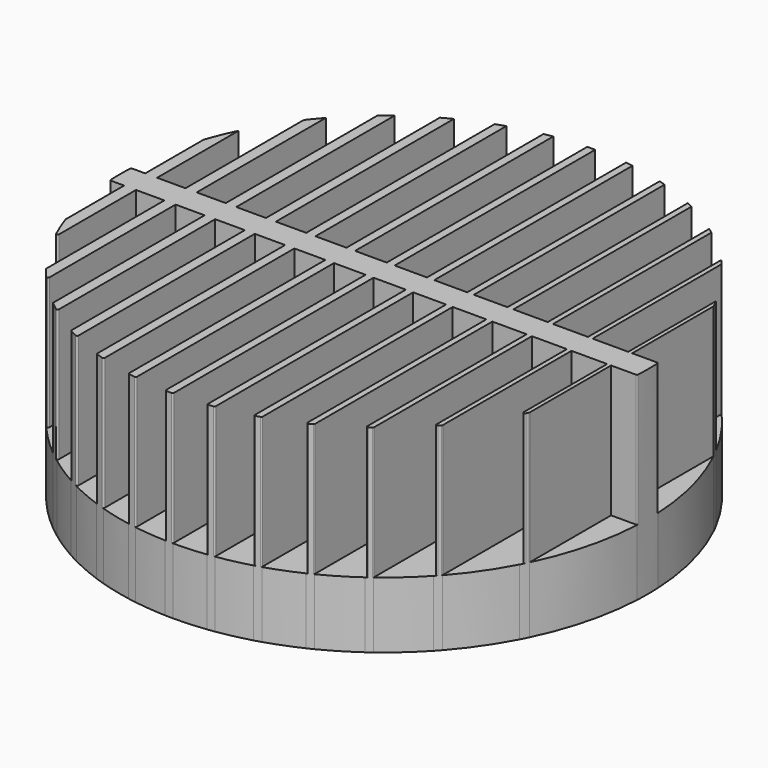
from build123d import *

# Parameters (mm, degrees)
F0_W         = 11
F0_H         = 5
F0_W_2       = 4.25
F0_W_3       = 3.25
F0_W_4       = 2.25
F0_W_5       = 3.5
F0_W_6       = 11.25
F0_W_7       = 11.5
F0_W_8       = 10.75
F0_W_9       = 4.5
F0_W_10      = 4
F0_W_11      = 3.75
F0_W_12      = 2
F0_W_13      = 13.5
F0_W_14      = 12.25
F0_W_15      = 1.75
F0_W_16      = 11.75
F0_W_17      = 13
F0_W_18      = 1.5
F0_W_19      = 2.5
F0_W_20      = 13.25
F0_W_21      = 12.75
F0_W_22      = 2.75
F0_W_23      = 12
F0_W_24      = 12.5
F0_W_25      = 3
F1_DEPTH     = 25
F2_DEPTH     = 75
F3_T1_DEPTH  = 50.2109984733
F3_T3_DEPTH  = 50.4269577712
F3_T5_DEPTH  = 53.3493232824
F3_T7_DEPTH  = 50.5880189906
F3_T9_DEPTH  = 52.5221366618
F3_T11_DEPTH = 50.7367983998
F3_T13_DEPTH = 52.0440371839
F3_T15_DEPTH = 50.8861030717
F3_T17_DEPTH = 51.7138805739
F3_T19_DEPTH = 51.0441499554
F3_T21_DEPTH = 51.4619110174
F3_T23_DEPTH = 51.2190561193
F3_T25_DEPTH = 51.2562853725
F3_T27_DEPTH = 51.4213816764
F3_T29_DEPTH = 51.0797077715
F3_T31_DEPTH = 51.6675925063
F3_T33_DEPTH = 50.921326192
F3_T35_DEPTH = 51.9875030892
F3_T37_DEPTH = 50.7731193512
F3_T39_DEPTH = 52.4451800761
F3_T41_DEPTH = 50.6275504684
F3_T43_DEPTH = 50.4743197485
F3_T45_DEPTH = 50.2878685654
F3_T47_DEPTH = 53.2195126732
F3_T49_DEPTH = 55.6061408631
F3_T51_DEPTH = 55.1888373464
F3_T53_DEPTH = 51.1948224465


# Not quite as in the source:
# - a fillet or chamfer that OpenCascade refuses, or shapes differently, is made with other operations: its cross-section is extruded or revolved along the edge and cut away or added


with BuildPart() as f1:
    # F0 (on Top) → F1 (new body)
    with BuildSketch(Plane.XY):
        with BuildLine():
            ThreePointArc((-99.8749217772, -5), (-98.1698653955, -19.0440943139), (-94.5, -32.7070328829))
            Line((-94.5, -32.7070328829), (-94.5, -5))
            Line((-94.5, -5), (-99.8749217772, -5))
        make_face()
        with BuildLine():
            Line((-94.5, -5), (-94.5, 0))
            Line((-94.5, 0), (-100, 0))
            ThreePointArc((-100, 0), (-99.9687255538, -2.5007821058), (-99.8749217772, -5))
            Line((-99.8749217772, -5), (-94.5, -5))
        make_face()
        with BuildLine():
            Line((-100, 0), (-94.5, 0))
            Line((-94.5, 0), (-94.5, 5))
            Line((-94.5, 5), (-99.8749217772, 5))
            ThreePointArc((-99.8749217772, 5), (-99.9687255538, 2.5007821058), (-100, 0))
        make_face()
        with BuildLine():
            Line((-94.5, 5), (-94.5, 32.7070328829))
            ThreePointArc((-94.5, 32.7070328829), (-98.1698653955, 19.0440943139), (-99.8749217772, 5))
            Line((-99.8749217772, 5), (-94.5, 5))
        make_face()
        with BuildLine():
            ThreePointArc((-15, -98.8685996664), (-9.0163773723, -99.5926952094), (-3, -99.9549898704))
            Line((-3, -99.9549898704), (-3, -5))
            Line((-3, -5), (-15, -5))
            Line((-15, -5), (-15, -98.8685996664))
        make_face()
        with BuildLine():
            Line((-30, 5), (-30, 95.3939201417))
            ThreePointArc((-30, 95.3939201417), (-31.7554083414, 94.8240161619), (-33.5, 94.2218127612))
            Line((-33.5, 94.2218127612), (-33.5, 5))
            Line((-33.5, 5), (-30, 5))
        make_face()
        with BuildLine():
            Line((-3, 5), (-3, 99.9549898704))
            ThreePointArc((-3, 99.9549898704), (-9.0163773723, 99.5926952094), (-15, 98.8685996664))
            Line((-15, 98.8685996664), (-15, 5))
            Line((-15, 5), (-3, 5))
        make_face()
        with BuildLine():
            ThreePointArc((12.25, -99.2468513354), (13.6263125453, -99.067268088), (15, -98.8685996664))
            Line((15, -98.8685996664), (15, -5))
            Line((15, -5), (12.25, -5))
            Line((12.25, -5), (12.25, -99.2468513354))
        make_face()
        with Locations((-69.5, -2.5)):
            Rectangle(F0_W, F0_H)
        with BuildLine():
            Line((-18.25, 5), (-18.25, 98.3205853319))
            ThreePointArc((-18.25, 98.3205853319), (-24.1693394052, 97.0352669534), (-30, 95.3939201417))
            Line((-30, 95.3939201417), (-30, 5))
            Line((-30, 5), (-18.25, 5))
        make_face()
        with Locations((-77.125, -2.5)):
            Rectangle(F0_W_2, F0_H)
        with BuildLine():
            Line((45, 5), (45, 89.3028554975))
            ThreePointArc((45, 89.3028554975), (43.878438886, 89.859237705), (42.75, 90.4015348321))
            Line((42.75, 90.4015348321), (42.75, 5))
            Line((42.75, 5), (45, 5))
        make_face()
        with Locations((-16.625, 2.5)):
            Rectangle(F0_W_3, F0_H)
        with BuildLine():
            Line((42.75, 5), (42.75, 90.4015348321))
            ThreePointArc((42.75, 90.4015348321), (36.4605485802, 93.1162091004), (30, 95.3939201417))
            Line((30, 95.3939201417), (30, 5))
            Line((30, 5), (42.75, 5))
        make_face()
        with Locations((43.875, -2.5)):
            Rectangle(F0_W_4, F0_H)
        with Locations((-31.75, -2.5)):
            Rectangle(F0_W_5, F0_H)
        with Locations((-54.375, -2.5)):
            Rectangle(F0_W_6, F0_H)
        with BuildLine():
            Line((30, 5), (30, 95.3939201417))
            ThreePointArc((30, 95.3939201417), (28.752448826, 95.7773286666), (27.5, 96.1444226151))
            Line((27.5, 96.1444226151), (27.5, 5))
            Line((27.5, 5), (30, 5))
        make_face()
        with BuildLine():
            Line((15, 5), (15, 98.8685996664))
            ThreePointArc((15, 98.8685996664), (13.6263125453, 99.067268088), (12.25, 99.2468513354))
            Line((12.25, 99.2468513354), (12.25, 5))
            Line((12.25, 5), (15, 5))
        make_face()
        with Locations((-39.25, 2.5)):
            Rectangle(F0_W_7, F0_H)
        with Locations((-84.625, 2.5)):
            Rectangle(F0_W_8, F0_H)
        with BuildLine():
            ThreePointArc((-75, -66.1437827766), (-69.7053717305, -71.7018908531), (-64, -76.8374908492))
            Line((-64, -76.8374908492), (-64, -5))
            Line((-64, -5), (-75, -5))
            Line((-75, -5), (-75, -66.1437827766))
        make_face()
        with Locations((-92.25, -2.5)):
            Rectangle(F0_W_9, F0_H)
        with BuildLine():
            ThreePointArc((45, -89.3028554975), (51.6490187326, -85.6293107759), (58, -81.4616474177))
            Line((58, -81.4616474177), (58, -5))
            Line((58, -5), (45, -5))
            Line((45, -5), (45, -89.3028554975))
        make_face()
        with Locations((-62, -2.5)):
            Rectangle(F0_W_10, F0_H)
        with BuildLine():
            ThreePointArc((15, -98.8685996664), (21.2936090213, -97.7066129535), (27.5, -96.1444226151))
            Line((27.5, -96.1444226151), (27.5, -5))
            Line((27.5, -5), (15, -5))
            Line((15, -5), (15, -98.8685996664))
        make_face()
        with Locations((-46.875, -2.5)):
            Rectangle(F0_W_11, F0_H)
        with BuildLine():
            Line((73.25, 5), (73.25, 68.0767030635))
            ThreePointArc((73.25, 68.0767030635), (66.8911943193, 74.3341652441), (60, 80))
            Line((60, 80), (60, 5))
            Line((60, 5), (73.25, 5))
        make_face()
        with BuildLine():
            ThreePointArc((-18.25, -98.3205853319), (-16.6272578896, -98.6079829176), (-15, -98.8685996664))
            Line((-15, -98.8685996664), (-15, -5))
            Line((-15, -5), (-18.25, -5))
            Line((-18.25, -5), (-18.25, -98.3205853319))
        make_face()
        with Locations((59, 2.5)):
            Rectangle(F0_W_12, F0_H)
        with Locations((81.75, 2.5)):
            Rectangle(F0_W_13, F0_H)
        with BuildLine():
            ThreePointArc((88.5, -46.559102225), (89.262354285, -45.0802851311), (90, -43.5889894354))
            Line((90, -43.5889894354), (90, -5))
            Line((90, -5), (88.5, -5))
            Line((88.5, -5), (88.5, -46.559102225))
        make_face()
        with Locations((6.125, -2.5)):
            Rectangle(F0_W_14, F0_H)
        with BuildLine():
            ThreePointArc((0, -100), (6.1365652631, -99.811535239), (12.25, -99.2468513354))
            Line((12.25, -99.2468513354), (12.25, -5))
            Line((12.25, -5), (0, -5))
            Line((0, -5), (0, -100))
        make_face()
        with BuildLine():
            Line((0, 5), (0, 100))
            ThreePointArc((0, 100), (-1.5001688165, 99.9887468344), (-3, 99.9549898704))
            Line((-3, 99.9549898704), (-3, 5))
            Line((-3, 5), (0, 5))
        make_face()
        with BuildLine():
            ThreePointArc((90, -43.5889894354), (96.8782690101, -24.7911474848), (99.8749217772, -5))
            Line((99.8749217772, -5), (90, -5))
            Line((90, -5), (90, -43.5889894354))
        make_face()
        with Locations((74.125, 2.5)):
            Rectangle(F0_W_15, F0_H)
        with BuildLine():
            Line((-79.25, 5), (-79.25, 60.9871912782))
            ThreePointArc((-79.25, 60.9871912782), (-85.0709408778, 52.5636282819), (-90, 43.5889894354))
            Line((-90, 43.5889894354), (-90, 5))
            Line((-90, 5), (-79.25, 5))
        make_face()
        with BuildLine():
            ThreePointArc((-64, -76.8374908492), (-62.0201609643, -78.4442453847), (-60, -80))
            Line((-60, -80), (-60, -5))
            Line((-60, -5), (-64, -5))
            Line((-64, -5), (-64, -76.8374908492))
        make_face()
        with BuildLine():
            Line((-48.75, 5), (-48.75, 87.3122986755))
            ThreePointArc((-48.75, 87.3122986755), (-54.4977802574, 83.845047242), (-60, 80))
            Line((-60, 80), (-60, 5))
            Line((-60, 5), (-48.75, 5))
        make_face()
        with BuildLine():
            ThreePointArc((42.75, -90.4015348321), (43.878438886, -89.859237705), (45, -89.3028554975))
            Line((45, -89.3028554975), (45, -5))
            Line((45, -5), (42.75, -5))
            Line((42.75, -5), (42.75, -90.4015348321))
        make_face()
        with BuildLine():
            ThreePointArc((60, -80), (66.8911943193, -74.3341652441), (73.25, -68.0767030635))
            Line((73.25, -68.0767030635), (73.25, -5))
            Line((73.25, -5), (60, -5))
            Line((60, -5), (60, -80))
        make_face()
        with Locations((-62, 2.5)):
            Rectangle(F0_W_10, F0_H)
        with Locations((-24.125, -2.5)):
            Rectangle(F0_W_16, F0_H)
        with BuildLine():
            ThreePointArc((58, -81.4616474177), (59.0045261255, -80.7370168925), (60, -80))
            Line((60, -80), (60, -5))
            Line((60, -5), (58, -5))
            Line((58, -5), (58, -81.4616474177))
        make_face()
        with BuildLine():
            ThreePointArc((-60, -80), (-54.4977802574, -83.845047242), (-48.75, -87.3122986755))
            Line((-48.75, -87.3122986755), (-48.75, -5))
            Line((-48.75, -5), (-60, -5))
            Line((-60, -5), (-60, -80))
        make_face()
        with Locations((51.5, -2.5)):
            Rectangle(F0_W_17, F0_H)
        with BuildLine():
            Line((27.5, 5), (27.5, 96.1444226151))
            ThreePointArc((27.5, 96.1444226151), (21.2936090213, 97.7066129535), (15, 98.8685996664))
            Line((15, 98.8685996664), (15, 5))
            Line((15, 5), (27.5, 5))
        make_face()
        with Locations((89.25, -2.5)):
            Rectangle(F0_W_18, F0_H)
        with BuildLine():
            Line((-75, 5), (-75, 66.1437827766))
            ThreePointArc((-75, 66.1437827766), (-77.1680842964, 63.6009965805), (-79.25, 60.9871912782))
            Line((-79.25, 60.9871912782), (-79.25, 5))
            Line((-79.25, 5), (-75, 5))
        make_face()
        with Locations((-39.25, -2.5)):
            Rectangle(F0_W_7, F0_H)
        with BuildLine():
            ThreePointArc((-94.5, -32.7070328829), (-92.410317306, -38.2143069464), (-90, -43.5889894354))
            Line((-90, -43.5889894354), (-90, -5))
            Line((-90, -5), (-94.5, -5))
            Line((-94.5, -5), (-94.5, -32.7070328829))
        make_face()
        with Locations((74.125, -2.5)):
            Rectangle(F0_W_15, F0_H)
        with Locations((28.75, -2.5)):
            Rectangle(F0_W_19, F0_H)
        with Locations((66.625, 2.5)):
            Rectangle(F0_W_20, F0_H)
        with Locations((-54.375, 2.5)):
            Rectangle(F0_W_6, F0_H)
        with BuildLine():
            ThreePointArc((-33.5, -94.2218127612), (-31.7554083414, -94.8240161619), (-30, -95.3939201417))
            Line((-30, -95.3939201417), (-30, -5))
            Line((-30, -5), (-33.5, -5))
            Line((-33.5, -5), (-33.5, -94.2218127612))
        make_face()
        with Locations((36.375, -2.5)):
            Rectangle(F0_W_21, F0_H)
        with Locations((66.625, -2.5)):
            Rectangle(F0_W_20, F0_H)
        with Locations((59, -2.5)):
            Rectangle(F0_W_12, F0_H)
        with BuildLine():
            Line((60, 5), (60, 80))
            ThreePointArc((60, 80), (59.0045261255, 80.7370168925), (58, 81.4616474177))
            Line((58, 81.4616474177), (58, 5))
            Line((58, 5), (60, 5))
        make_face()
        with Locations((43.875, 2.5)):
            Rectangle(F0_W_4, F0_H)
        with BuildLine():
            ThreePointArc((-45, -89.3028554975), (-39.3269822786, -91.942310526), (-33.5, -94.2218127612))
            Line((-33.5, -94.2218127612), (-33.5, -5))
            Line((-33.5, -5), (-45, -5))
            Line((-45, -5), (-45, -89.3028554975))
        make_face()
        with Locations((-46.875, 2.5)):
            Rectangle(F0_W_11, F0_H)
        with BuildLine():
            Line((-60, 5), (-60, 80))
            ThreePointArc((-60, 80), (-62.0201609643, 78.4442453847), (-64, 76.8374908492))
            Line((-64, 76.8374908492), (-64, 5))
            Line((-64, 5), (-60, 5))
        make_face()
        with BuildLine():
            ThreePointArc((-90, -43.5889894354), (-85.0709408778, -52.5636282819), (-79.25, -60.9871912782))
            Line((-79.25, -60.9871912782), (-79.25, -5))
            Line((-79.25, -5), (-90, -5))
            Line((-90, -5), (-90, -43.5889894354))
        make_face()
        with Locations((-16.625, -2.5)):
            Rectangle(F0_W_3, F0_H)
        with BuildLine():
            Line((12.25, 5), (12.25, 99.2468513354))
            ThreePointArc((12.25, 99.2468513354), (6.1365652631, 99.811535239), (0, 100))
            Line((0, 100), (0, 5))
            Line((0, 5), (12.25, 5))
        make_face()
        with BuildLine():
            Line((90, 5), (99.8749217772, 5))
            ThreePointArc((99.8749217772, 5), (96.8782690101, 24.7911474848), (90, 43.5889894354))
            Line((90, 43.5889894354), (90, 5))
        make_face()
        with Locations((-84.625, -2.5)):
            Rectangle(F0_W_8, F0_H)
        with Locations((-69.5, 2.5)):
            Rectangle(F0_W, F0_H)
        with BuildLine():
            ThreePointArc((27.5, -96.1444226151), (28.752448826, -95.7773286666), (30, -95.3939201417))
            Line((30, -95.3939201417), (30, -5))
            Line((30, -5), (27.5, -5))
            Line((27.5, -5), (27.5, -96.1444226151))
        make_face()
        with BuildLine():
            ThreePointArc((-48.75, -87.3122986755), (-46.8855649866, -88.3274804117), (-45, -89.3028554975))
            Line((-45, -89.3028554975), (-45, -5))
            Line((-45, -5), (-48.75, -5))
            Line((-48.75, -5), (-48.75, -87.3122986755))
        make_face()
        with BuildLine():
            Line((90, 5), (90, 43.5889894354))
            ThreePointArc((90, 43.5889894354), (89.262354285, 45.0802851311), (88.5, 46.559102225))
            Line((88.5, 46.559102225), (88.5, 5))
            Line((88.5, 5), (90, 5))
        make_face()
        with Locations((-77.125, 2.5)):
            Rectangle(F0_W_2, F0_H)
        with Locations((13.625, 2.5)):
            Rectangle(F0_W_22, F0_H)
        with BuildLine():
            Line((-33.5, 5), (-33.5, 94.2218127612))
            ThreePointArc((-33.5, 94.2218127612), (-39.3269822786, 91.942310526), (-45, 89.3028554975))
            Line((-45, 89.3028554975), (-45, 5))
            Line((-45, 5), (-33.5, 5))
        make_face()
        with Locations((-24.125, 2.5)):
            Rectangle(F0_W_16, F0_H)
        with Locations((-9, -2.5)):
            Rectangle(F0_W_23, F0_H)
        with Locations((21.25, -2.5)):
            Rectangle(F0_W_24, F0_H)
        with BuildLine():
            Line((-15, 5), (-15, 98.8685996664))
            ThreePointArc((-15, 98.8685996664), (-16.6272578896, 98.6079829176), (-18.25, 98.3205853319))
            Line((-18.25, 98.3205853319), (-18.25, 5))
            Line((-18.25, 5), (-15, 5))
        make_face()
        with BuildLine():
            ThreePointArc((99.8749217772, -5), (99.9687255538, -2.5007821058), (100, 0))
            Line((100, 0), (90, 0))
            Line((90, 0), (90, -5))
            Line((90, -5), (99.8749217772, -5))
        make_face()
        with Locations((36.375, 2.5)):
            Rectangle(F0_W_21, F0_H)
        with BuildLine():
            ThreePointArc((75, -66.1437827766), (82.3343939558, -56.7542736005), (88.5, -46.559102225))
            Line((88.5, -46.559102225), (88.5, -5))
            Line((88.5, -5), (75, -5))
            Line((75, -5), (75, -66.1437827766))
        make_face()
        with Locations((6.125, 2.5)):
            Rectangle(F0_W_14, F0_H)
        with Locations((81.75, -2.5)):
            Rectangle(F0_W_13, F0_H)
        with Locations((13.625, -2.5)):
            Rectangle(F0_W_22, F0_H)
        with BuildLine():
            Line((90, 0), (100, 0))
            ThreePointArc((100, 0), (99.9687255538, 2.5007821058), (99.8749217772, 5))
            Line((99.8749217772, 5), (90, 5))
            Line((90, 5), (90, 0))
        make_face()
        with Locations((28.75, 2.5)):
            Rectangle(F0_W_19, F0_H)
        with BuildLine():
            Line((-64, 5), (-64, 76.8374908492))
            ThreePointArc((-64, 76.8374908492), (-69.7053717305, 71.7018908531), (-75, 66.1437827766))
            Line((-75, 66.1437827766), (-75, 5))
            Line((-75, 5), (-64, 5))
        make_face()
        with Locations((-92.25, 2.5)):
            Rectangle(F0_W_9, F0_H)
        with BuildLine():
            Line((88.5, 5), (88.5, 46.559102225))
            ThreePointArc((88.5, 46.559102225), (82.3343939558, 56.7542736005), (75, 66.1437827766))
            Line((75, 66.1437827766), (75, 5))
            Line((75, 5), (88.5, 5))
        make_face()
        with BuildLine():
            Line((-45, 5), (-45, 89.3028554975))
            ThreePointArc((-45, 89.3028554975), (-46.8855649866, 88.3274804117), (-48.75, 87.3122986755))
            Line((-48.75, 87.3122986755), (-48.75, 5))
            Line((-48.75, 5), (-45, 5))
        make_face()
        with BuildLine():
            ThreePointArc((30, -95.3939201417), (36.4605485802, -93.1162091004), (42.75, -90.4015348321))
            Line((42.75, -90.4015348321), (42.75, -5))
            Line((42.75, -5), (30, -5))
            Line((30, -5), (30, -95.3939201417))
        make_face()
        with Locations((-31.75, 2.5)):
            Rectangle(F0_W_5, F0_H)
        with BuildLine():
            ThreePointArc((-79.25, -60.9871912782), (-77.1680842964, -63.6009965805), (-75, -66.1437827766))
            Line((-75, -66.1437827766), (-75, -5))
            Line((-75, -5), (-79.25, -5))
            Line((-79.25, -5), (-79.25, -60.9871912782))
        make_face()
        with BuildLine():
            Line((-90, 5), (-90, 43.5889894354))
            ThreePointArc((-90, 43.5889894354), (-92.410317306, 38.2143069464), (-94.5, 32.7070328829))
            Line((-94.5, 32.7070328829), (-94.5, 5))
            Line((-94.5, 5), (-90, 5))
        make_face()
        with Locations((21.25, 2.5)):
            Rectangle(F0_W_24, F0_H)
        with BuildLine():
            Line((58, 5), (58, 81.4616474177))
            ThreePointArc((58, 81.4616474177), (51.6490187326, 85.6293107759), (45, 89.3028554975))
            Line((45, 89.3028554975), (45, 5))
            Line((45, 5), (58, 5))
        make_face()
        with Locations((89.25, 2.5)):
            Rectangle(F0_W_18, F0_H)
        with BuildLine():
            Line((75, 5), (75, 66.1437827766))
            ThreePointArc((75, 66.1437827766), (74.1313002058, 67.1159469112), (73.25, 68.0767030635))
            Line((73.25, 68.0767030635), (73.25, 5))
            Line((73.25, 5), (75, 5))
        make_face()
        with Locations((-9, 2.5)):
            Rectangle(F0_W_23, F0_H)
        with BuildLine():
            ThreePointArc((-30, -95.3939201417), (-24.1693394052, -97.0352669534), (-18.25, -98.3205853319))
            Line((-18.25, -98.3205853319), (-18.25, -5))
            Line((-18.25, -5), (-30, -5))
            Line((-30, -5), (-30, -95.3939201417))
        make_face()
        with BuildLine():
            ThreePointArc((73.25, -68.0767030635), (74.1313002058, -67.1159469112), (75, -66.1437827766))
            Line((75, -66.1437827766), (75, -5))
            Line((75, -5), (73.25, -5))
            Line((73.25, -5), (73.25, -68.0767030635))
        make_face()
        with BuildLine():
            ThreePointArc((-3, -99.9549898704), (-1.5001688165, -99.9887468344), (0, -100))
            Line((0, -100), (0, -5))
            Line((0, -5), (-3, -5))
            Line((-3, -5), (-3, -99.9549898704))
        make_face()
        with Locations((51.5, 2.5)):
            Rectangle(F0_W_17, F0_H)
        with Locations((-1.5, 2.5)):
            Rectangle(F0_W_25, F0_H)
        with Locations((-1.5, -2.5)):
            Rectangle(F0_W_25, F0_H)
    extrude(amount=F1_DEPTH)

    # F0 (on Top) → F2 (join)
    with BuildSketch(Plane.XY):
        with BuildLine():
            ThreePointArc((99.8749217772, -5), (99.9687255538, -2.5007821058), (100, 0))
            Line((100, 0), (90, 0))
            Line((90, 0), (90, -5))
            Line((90, -5), (99.8749217772, -5))
        make_face()
        with BuildLine():
            Line((90, 0), (100, 0))
            ThreePointArc((100, 0), (99.9687255538, 2.5007821058), (99.8749217772, 5))
            Line((99.8749217772, 5), (90, 5))
            Line((90, 5), (90, 0))
        make_face()
        with Locations((89.25, 2.5)):
            Rectangle(F0_W_18, F0_H)
        with BuildLine():
            Line((90, 5), (90, 43.5889894354))
            ThreePointArc((90, 43.5889894354), (89.262354285, 45.0802851311), (88.5, 46.559102225))
            Line((88.5, 46.559102225), (88.5, 5))
            Line((88.5, 5), (90, 5))
        make_face()
        with Locations((81.75, 2.5)):
            Rectangle(F0_W_13, F0_H)
        with Locations((81.75, -2.5)):
            Rectangle(F0_W_13, F0_H)
        with Locations((89.25, -2.5)):
            Rectangle(F0_W_18, F0_H)
        with BuildLine():
            ThreePointArc((88.5, -46.559102225), (89.262354285, -45.0802851311), (90, -43.5889894354))
            Line((90, -43.5889894354), (90, -5))
            Line((90, -5), (88.5, -5))
            Line((88.5, -5), (88.5, -46.559102225))
        make_face()
        with Locations((74.125, -2.5)):
            Rectangle(F0_W_15, F0_H)
        with BuildLine():
            ThreePointArc((73.25, -68.0767030635), (74.1313002058, -67.1159469112), (75, -66.1437827766))
            Line((75, -66.1437827766), (75, -5))
            Line((75, -5), (73.25, -5))
            Line((73.25, -5), (73.25, -68.0767030635))
        make_face()
        with Locations((74.125, 2.5)):
            Rectangle(F0_W_15, F0_H)
        with Locations((66.625, 2.5)):
            Rectangle(F0_W_20, F0_H)
        with Locations((66.625, -2.5)):
            Rectangle(F0_W_20, F0_H)
        with BuildLine():
            Line((75, 5), (75, 66.1437827766))
            ThreePointArc((75, 66.1437827766), (74.1313002058, 67.1159469112), (73.25, 68.0767030635))
            Line((73.25, 68.0767030635), (73.25, 5))
            Line((73.25, 5), (75, 5))
        make_face()
        with Locations((59, 2.5)):
            Rectangle(F0_W_12, F0_H)
        with BuildLine():
            Line((60, 5), (60, 80))
            ThreePointArc((60, 80), (59.0045261255, 80.7370168925), (58, 81.4616474177))
            Line((58, 81.4616474177), (58, 5))
            Line((58, 5), (60, 5))
        make_face()
        with Locations((51.5, 2.5)):
            Rectangle(F0_W_17, F0_H)
        with Locations((51.5, -2.5)):
            Rectangle(F0_W_17, F0_H)
        with Locations((59, -2.5)):
            Rectangle(F0_W_12, F0_H)
        with BuildLine():
            ThreePointArc((58, -81.4616474177), (59.0045261255, -80.7370168925), (60, -80))
            Line((60, -80), (60, -5))
            Line((60, -5), (58, -5))
            Line((58, -5), (58, -81.4616474177))
        make_face()
        with Locations((43.875, -2.5)):
            Rectangle(F0_W_4, F0_H)
        with Locations((43.875, 2.5)):
            Rectangle(F0_W_4, F0_H)
        with BuildLine():
            Line((45, 5), (45, 89.3028554975))
            ThreePointArc((45, 89.3028554975), (43.878438886, 89.859237705), (42.75, 90.4015348321))
            Line((42.75, 90.4015348321), (42.75, 5))
            Line((42.75, 5), (45, 5))
        make_face()
        with Locations((36.375, 2.5)):
            Rectangle(F0_W_21, F0_H)
        with Locations((36.375, -2.5)):
            Rectangle(F0_W_21, F0_H)
        with BuildLine():
            ThreePointArc((42.75, -90.4015348321), (43.878438886, -89.859237705), (45, -89.3028554975))
            Line((45, -89.3028554975), (45, -5))
            Line((45, -5), (42.75, -5))
            Line((42.75, -5), (42.75, -90.4015348321))
        make_face()
        with Locations((28.75, -2.5)):
            Rectangle(F0_W_19, F0_H)
        with Locations((28.75, 2.5)):
            Rectangle(F0_W_19, F0_H)
        with Locations((21.25, 2.5)):
            Rectangle(F0_W_24, F0_H)
        with Locations((21.25, -2.5)):
            Rectangle(F0_W_24, F0_H)
        with BuildLine():
            Line((30, 5), (30, 95.3939201417))
            ThreePointArc((30, 95.3939201417), (28.752448826, 95.7773286666), (27.5, 96.1444226151))
            Line((27.5, 96.1444226151), (27.5, 5))
            Line((27.5, 5), (30, 5))
        make_face()
        with BuildLine():
            ThreePointArc((27.5, -96.1444226151), (28.752448826, -95.7773286666), (30, -95.3939201417))
            Line((30, -95.3939201417), (30, -5))
            Line((30, -5), (27.5, -5))
            Line((27.5, -5), (27.5, -96.1444226151))
        make_face()
        with Locations((13.625, -2.5)):
            Rectangle(F0_W_22, F0_H)
        with Locations((13.625, 2.5)):
            Rectangle(F0_W_22, F0_H)
        with Locations((6.125, 2.5)):
            Rectangle(F0_W_14, F0_H)
        with Locations((6.125, -2.5)):
            Rectangle(F0_W_14, F0_H)
        with BuildLine():
            Line((15, 5), (15, 98.8685996664))
            ThreePointArc((15, 98.8685996664), (13.6263125453, 99.067268088), (12.25, 99.2468513354))
            Line((12.25, 99.2468513354), (12.25, 5))
            Line((12.25, 5), (15, 5))
        make_face()
        with BuildLine():
            ThreePointArc((12.25, -99.2468513354), (13.6263125453, -99.067268088), (15, -98.8685996664))
            Line((15, -98.8685996664), (15, -5))
            Line((15, -5), (12.25, -5))
            Line((12.25, -5), (12.25, -99.2468513354))
        make_face()
        with Locations((-1.5, -2.5)):
            Rectangle(F0_W_25, F0_H)
        with Locations((-9, -2.5)):
            Rectangle(F0_W_23, F0_H)
        with Locations((-9, 2.5)):
            Rectangle(F0_W_23, F0_H)
        with Locations((-1.5, 2.5)):
            Rectangle(F0_W_25, F0_H)
        with BuildLine():
            Line((0, 5), (0, 100))
            ThreePointArc((0, 100), (-1.5001688165, 99.9887468344), (-3, 99.9549898704))
            Line((-3, 99.9549898704), (-3, 5))
            Line((-3, 5), (0, 5))
        make_face()
        with BuildLine():
            ThreePointArc((-3, -99.9549898704), (-1.5001688165, -99.9887468344), (0, -100))
            Line((0, -100), (0, -5))
            Line((0, -5), (-3, -5))
            Line((-3, -5), (-3, -99.9549898704))
        make_face()
        with Locations((-16.625, -2.5)):
            Rectangle(F0_W_3, F0_H)
        with BuildLine():
            ThreePointArc((-18.25, -98.3205853319), (-16.6272578896, -98.6079829176), (-15, -98.8685996664))
            Line((-15, -98.8685996664), (-15, -5))
            Line((-15, -5), (-18.25, -5))
            Line((-18.25, -5), (-18.25, -98.3205853319))
        make_face()
        with Locations((-24.125, -2.5)):
            Rectangle(F0_W_16, F0_H)
        with Locations((-24.125, 2.5)):
            Rectangle(F0_W_16, F0_H)
        with Locations((-16.625, 2.5)):
            Rectangle(F0_W_3, F0_H)
        with BuildLine():
            Line((-15, 5), (-15, 98.8685996664))
            ThreePointArc((-15, 98.8685996664), (-16.6272578896, 98.6079829176), (-18.25, 98.3205853319))
            Line((-18.25, 98.3205853319), (-18.25, 5))
            Line((-18.25, 5), (-15, 5))
        make_face()
        with BuildLine():
            Line((-30, 5), (-30, 95.3939201417))
            ThreePointArc((-30, 95.3939201417), (-31.7554083414, 94.8240161619), (-33.5, 94.2218127612))
            Line((-33.5, 94.2218127612), (-33.5, 5))
            Line((-33.5, 5), (-30, 5))
        make_face()
        with Locations((-31.75, 2.5)):
            Rectangle(F0_W_5, F0_H)
        with Locations((-39.25, 2.5)):
            Rectangle(F0_W_7, F0_H)
        with Locations((-39.25, -2.5)):
            Rectangle(F0_W_7, F0_H)
        with Locations((-31.75, -2.5)):
            Rectangle(F0_W_5, F0_H)
        with BuildLine():
            ThreePointArc((-33.5, -94.2218127612), (-31.7554083414, -94.8240161619), (-30, -95.3939201417))
            Line((-30, -95.3939201417), (-30, -5))
            Line((-30, -5), (-33.5, -5))
            Line((-33.5, -5), (-33.5, -94.2218127612))
        make_face()
        with Locations((-46.875, -2.5)):
            Rectangle(F0_W_11, F0_H)
        with BuildLine():
            ThreePointArc((-48.75, -87.3122986755), (-46.8855649866, -88.3274804117), (-45, -89.3028554975))
            Line((-45, -89.3028554975), (-45, -5))
            Line((-45, -5), (-48.75, -5))
            Line((-48.75, -5), (-48.75, -87.3122986755))
        make_face()
        with Locations((-54.375, -2.5)):
            Rectangle(F0_W_6, F0_H)
        with Locations((-46.875, 2.5)):
            Rectangle(F0_W_11, F0_H)
        with BuildLine():
            Line((-45, 5), (-45, 89.3028554975))
            ThreePointArc((-45, 89.3028554975), (-46.8855649866, 88.3274804117), (-48.75, 87.3122986755))
            Line((-48.75, 87.3122986755), (-48.75, 5))
            Line((-48.75, 5), (-45, 5))
        make_face()
        with Locations((-54.375, 2.5)):
            Rectangle(F0_W_6, F0_H)
        with Locations((-62, 2.5)):
            Rectangle(F0_W_10, F0_H)
        with Locations((-69.5, 2.5)):
            Rectangle(F0_W, F0_H)
        with Locations((-62, -2.5)):
            Rectangle(F0_W_10, F0_H)
        with BuildLine():
            ThreePointArc((-64, -76.8374908492), (-62.0201609643, -78.4442453847), (-60, -80))
            Line((-60, -80), (-60, -5))
            Line((-60, -5), (-64, -5))
            Line((-64, -5), (-64, -76.8374908492))
        make_face()
        with BuildLine():
            Line((-60, 5), (-60, 80))
            ThreePointArc((-60, 80), (-62.0201609643, 78.4442453847), (-64, 76.8374908492))
            Line((-64, 76.8374908492), (-64, 5))
            Line((-64, 5), (-60, 5))
        make_face()
        with Locations((-77.125, 2.5)):
            Rectangle(F0_W_2, F0_H)
        with Locations((-84.625, 2.5)):
            Rectangle(F0_W_8, F0_H)
        with Locations((-69.5, -2.5)):
            Rectangle(F0_W, F0_H)
        with Locations((-77.125, -2.5)):
            Rectangle(F0_W_2, F0_H)
        with BuildLine():
            ThreePointArc((-79.25, -60.9871912782), (-77.1680842964, -63.6009965805), (-75, -66.1437827766))
            Line((-75, -66.1437827766), (-75, -5))
            Line((-75, -5), (-79.25, -5))
            Line((-79.25, -5), (-79.25, -60.9871912782))
        make_face()
        with BuildLine():
            Line((-75, 5), (-75, 66.1437827766))
            ThreePointArc((-75, 66.1437827766), (-77.1680842964, 63.6009965805), (-79.25, 60.9871912782))
            Line((-79.25, 60.9871912782), (-79.25, 5))
            Line((-79.25, 5), (-75, 5))
        make_face()
        with Locations((-84.625, -2.5)):
            Rectangle(F0_W_8, F0_H)
        with Locations((-92.25, 2.5)):
            Rectangle(F0_W_9, F0_H)
        with BuildLine():
            Line((-90, 5), (-90, 43.5889894354))
            ThreePointArc((-90, 43.5889894354), (-92.410317306, 38.2143069464), (-94.5, 32.7070328829))
            Line((-94.5, 32.7070328829), (-94.5, 5))
            Line((-94.5, 5), (-90, 5))
        make_face()
        with BuildLine():
            Line((-100, 0), (-94.5, 0))
            Line((-94.5, 0), (-94.5, 5))
            Line((-94.5, 5), (-99.8749217772, 5))
            ThreePointArc((-99.8749217772, 5), (-99.9687255538, 2.5007821058), (-100, 0))
        make_face()
        with BuildLine():
            Line((-94.5, -5), (-94.5, 0))
            Line((-94.5, 0), (-100, 0))
            ThreePointArc((-100, 0), (-99.9687255538, -2.5007821058), (-99.8749217772, -5))
            Line((-99.8749217772, -5), (-94.5, -5))
        make_face()
        with Locations((-92.25, -2.5)):
            Rectangle(F0_W_9, F0_H)
        with BuildLine():
            ThreePointArc((-94.5, -32.7070328829), (-92.410317306, -38.2143069464), (-90, -43.5889894354))
            Line((-90, -43.5889894354), (-90, -5))
            Line((-90, -5), (-94.5, -5))
            Line((-94.5, -5), (-94.5, -32.7070328829))
        make_face()
    extrude(amount=F2_DEPTH)

    # F3: fillet of radius 0.5 on 30 edges, made by hand

    # F3_s2 → F3_t1 (cut)
    with BuildSketch(Plane.XY.offset(25)):
        with BuildLine():
            ThreePointArc((-94.472361809, -32.7867786496), (-94.493042039, -32.7059684458), (-94.5, -32.6228447564))
            Line((-94.5, -32.6228447564), (-94.5, -32.7070328829))
            ThreePointArc((-94.5, -32.7070328829), (-94.4861893176, -32.7469086821), (-94.472361809, -32.7867786496))
        make_face()
    extrude(amount=F3_T1_DEPTH, mode=Mode.SUBTRACT)

    # F3_s4 → F3_t3 (cut)
    with BuildSketch(Plane.XY.offset(25)):
        with BuildLine():
            ThreePointArc((-79.1457286432, -61.122447902), (-79.223214709, -60.9782910408), (-79.25, -60.8168356625))
            Line((-79.25, -60.8168356625), (-79.25, -60.9871912782))
            ThreePointArc((-79.25, -60.9871912782), (-79.197893196, -61.0548418498), (-79.1457286432, -61.122447902))
        make_face()
    extrude(amount=F3_T3_DEPTH, mode=Mode.SUBTRACT)

    # F3_s6 → F3_t5 (cut)
    with BuildSketch(Plane.XY.offset(25)):
        with BuildLine():
            ThreePointArc((-75.8793969849, -65.1330723458), (-75.3263602759, -65.2762878285), (-75, -64.8074069841))
            Line((-75, -64.8074069841), (-75, -66.1437827766))
            ThreePointArc((-75, -66.1437827766), (-75.4413911094, -65.6399002701), (-75.8793969849, -65.1330723458))
        make_face()
    extrude(amount=F3_T5_DEPTH, mode=Mode.SUBTRACT)

    # F3_s8 → F3_t7 (cut)
    with BuildSketch(Plane.XY.offset(25)):
        with BuildLine():
            ThreePointArc((-63.8190954774, -76.9878110641), (-63.9525194685, -76.8155363703), (-64, -76.6028720088))
            Line((-64, -76.6028720088), (-64, -76.8374908492))
            ThreePointArc((-64, -76.8374908492), (-63.9095919343, -76.9127041443), (-63.8190954774, -76.9878110641))
        make_face()
    extrude(amount=F3_T7_DEPTH, mode=Mode.SUBTRACT)

    # F3_s10 → F3_t9 (cut)
    with BuildSketch(Plane.XY.offset(25)):
        with BuildLine():
            ThreePointArc((-60.8040201005, -79.3906237513), (-60.2786519147, -79.4420064722), (-60, -78.9936706325))
            Line((-60, -78.9936706325), (-60, -80))
            ThreePointArc((-60, -80), (-60.4027785202, -79.6963258064), (-60.8040201005, -79.3906237513))
        make_face()
    extrude(amount=F3_T9_DEPTH, mode=Mode.SUBTRACT)

    # F3_s12 → F3_t11 (cut)
    with BuildSketch(Plane.XY.offset(25)):
        with BuildLine():
            ThreePointArc((-48.4924623116, -87.4555950123), (-48.6808312638, -87.2720578935), (-48.75, -87.0183170373))
            Line((-48.75, -87.0183170373), (-48.75, -87.3122986755))
            ThreePointArc((-48.75, -87.3122986755), (-48.6212839461, -87.3840417207), (-48.4924623116, -87.4555950123))
        make_face()
    extrude(amount=F3_T11_DEPTH, mode=Mode.SUBTRACT)

    # F3_s14 → F3_t13 (cut)
    with BuildSketch(Plane.XY.offset(25)):
        with BuildLine():
            ThreePointArc((-45.7286432161, -88.9319469573), (-45.2395404139, -88.9140902263), (-45, -88.4872872225))
            Line((-45, -88.4872872225), (-45, -89.3028554975))
            ThreePointArc((-45, -89.3028554975), (-45.364700685, -89.1181459174), (-45.7286432161, -88.9319469573))
        make_face()
    extrude(amount=F3_T13_DEPTH, mode=Mode.SUBTRACT)

    # F3_s16 → F3_t15 (cut)
    with BuildSketch(Plane.XY.offset(25)):
        with BuildLine():
            ThreePointArc((-33.1658291457, -94.3399585387), (-33.4079917725, -94.1572963103), (-33.5, -93.868258746))
            Line((-33.5, -93.868258746), (-33.5, -94.2218127612))
            ThreePointArc((-33.5, -94.2218127612), (-33.3329669176, -94.2810337049), (-33.1658291457, -94.3399585387))
        make_face()
    extrude(amount=F3_T15_DEPTH, mode=Mode.SUBTRACT)

    # F3_s18 → F3_t17 (cut)
    with BuildSketch(Plane.XY.offset(25)):
        with BuildLine():
            ThreePointArc((-30.6532663317, -95.1860140105), (-30.2055795233, -95.114208405), (-30, -94.7100839404))
            Line((-30, -94.7100839404), (-30, -95.3939201417))
            ThreePointArc((-30, -95.3939201417), (-30.3268113295, -95.290526888), (-30.6532663317, -95.1860140105))
        make_face()
    extrude(amount=F3_T17_DEPTH, mode=Mode.SUBTRACT)

    # F3_s20 → F3_t19 (cut)
    with BuildSketch(Plane.XY.offset(25)):
        with BuildLine():
            ThreePointArc((-17.8391959799, -98.3959505609), (-18.1337955119, -98.2244407834), (-18.25, -97.9039708081))
            Line((-18.25, -97.9039708081), (-18.25, -98.3205853319))
            ThreePointArc((-18.25, -98.3205853319), (-18.0446373363, -98.3584824171), (-17.8391959799, -98.3959505609))
        make_face()
    extrude(amount=F3_T19_DEPTH, mode=Mode.SUBTRACT)

    # F3_s22 → F3_t21 (cut)
    with BuildSketch(Plane.XY.offset(25)):
        with BuildLine():
            ThreePointArc((-15.5778894472, -98.7791949773), (-15.1751498219, -98.6653942034), (-15, -98.2852990024))
            Line((-15, -98.2852990024), (-15, -98.8685996664))
            ThreePointArc((-15, -98.8685996664), (-15.2890100746, -98.8243197343), (-15.5778894472, -98.7791949773))
        make_face()
    extrude(amount=F3_T21_DEPTH, mode=Mode.SUBTRACT)

    # F3_s24 → F3_t23 (cut)
    with BuildSketch(Plane.XY.offset(25)):
        with BuildLine():
            ThreePointArc((-2.5125628141, -99.9684301573), (-2.8579674615, -99.8176715158), (-3, -99.4685880065))
            Line((-3, -99.4685880065), (-3, -99.9549898704))
            ThreePointArc((-3, -99.9549898704), (-2.7562895993, -99.9620071209), (-2.5125628141, -99.9684301573))
        make_face()
    extrude(amount=F3_T23_DEPTH, mode=Mode.SUBTRACT)

    # F3_s26 → F3_t25 (cut)
    with BuildSketch(Plane.XY.offset(25)):
        with BuildLine():
            ThreePointArc((-0.5025125628, -99.9987373977), (-0.1473360533, -99.8531843132), (0, -99.4987437107))
            Line((0, -99.4987437107), (0, -100))
            ThreePointArc((0, -100), (-0.2512570745, -99.9996843489), (-0.5025125628, -99.9987373977))
        make_face()
    extrude(amount=F3_T25_DEPTH, mode=Mode.SUBTRACT)

    # F3_s28 → F3_t27 (cut)
    with BuildSketch(Plane.XY.offset(25)):
        with BuildLine():
            ThreePointArc((12.8140703518, -99.1755998269), (12.4198751569, -99.0552449135), (12.25, -98.6797218277))
            Line((12.25, -98.6797218277), (12.25, -99.2468513354))
            ThreePointArc((12.25, -99.2468513354), (12.5320858138, -99.2116264616), (12.8140703518, -99.1755998269))
        make_face()
    extrude(amount=F3_T27_DEPTH, mode=Mode.SUBTRACT)

    # F3_s30 → F3_t29 (cut)
    with BuildSketch(Plane.XY.offset(25)):
        with BuildLine():
            ThreePointArc((14.5728643216, -98.9324599182), (14.8784390049, -98.7645757078), (15, -98.4377976186))
            Line((15, -98.4377976186), (15, -98.8685996664))
            ThreePointArc((15, -98.8685996664), (14.786466636, -98.9007603834), (14.5728643216, -98.9324599182))
        make_face()
    extrude(amount=F3_T29_DEPTH, mode=Mode.SUBTRACT)

    # F3_s32 → F3_t31 (cut)
    with BuildSketch(Plane.XY.offset(25)):
        with BuildLine():
            ThreePointArc((28.1407035176, -95.9588495426), (27.7002932757, -95.8792750837), (27.5, -95.4790552949))
            Line((27.5, -95.4790552949), (27.5, -96.1444226151))
            ThreePointArc((27.5, -96.1444226151), (27.8205064894, -96.0521702965), (28.1407035176, -95.9588495426))
        make_face()
    extrude(amount=F3_T31_DEPTH, mode=Mode.SUBTRACT)

    # F3_s34 → F3_t33 (cut)
    with BuildSketch(Plane.XY.offset(25)):
        with BuildLine():
            ThreePointArc((29.648241206, -95.5038313022), (29.9025671391, -95.3228584295), (30, -95.0263121456))
            Line((30, -95.0263121456), (30, -95.3939201417))
            ThreePointArc((30, -95.3939201417), (29.8241712351, -95.4490377644), (29.648241206, -95.5038313022))
        make_face()
    extrude(amount=F3_T33_DEPTH, mode=Mode.SUBTRACT)

    # F3_s36 → F3_t35 (cut)
    with BuildSketch(Plane.XY.offset(25)):
        with BuildLine():
            ThreePointArc((43.4673366834, -90.0588176785), (42.9841695481, -90.0320022447), (42.75, -89.6085235901))
            Line((42.75, -89.6085235901), (42.75, -90.4015348321))
            ThreePointArc((42.75, -90.4015348321), (43.1090089188, -90.2308891126), (43.4673366834, -90.0588176785))
        make_face()
    extrude(amount=F3_T35_DEPTH, mode=Mode.SUBTRACT)

    # F3_s38 → F3_t37 (cut)
    with BuildSketch(Plane.XY.offset(25)):
        with BuildLine():
            ThreePointArc((44.7236180905, -89.4415897941), (44.925328723, -89.2572420312), (45, -88.9943818452))
            Line((45, -88.9943818452), (45, -89.3028554975))
            ThreePointArc((45, -89.3028554975), (44.8618626743, -89.372329484), (44.7236180905, -89.4415897941))
        make_face()
    extrude(amount=F3_T37_DEPTH, mode=Mode.SUBTRACT)

    # F3_s40 → F3_t39 (cut)
    with BuildSketch(Plane.XY.offset(25)):
        with BuildLine():
            ThreePointArc((58.7939698492, -80.8904760115), (58.2730472787, -80.9315485604), (58, -80.4860236314))
            Line((58, -80.4860236314), (58, -81.4616474177))
            ThreePointArc((58, -81.4616474177), (58.3976832373, -81.17703242), (58.7939698492, -80.8904760115))
        make_face()
    extrude(amount=F3_T39_DEPTH, mode=Mode.SUBTRACT)

    # F3_s42 → F3_t41 (cut)
    with BuildSketch(Plane.XY.offset(25)):
        with BuildLine():
            ThreePointArc((59.7989949749, -80.1503599493), (59.9469325942, -79.9737760693), (60, -79.7496081495))
            Line((60, -79.7496081495), (60, -80))
            ThreePointArc((60, -80), (59.8995446667, -80.0752430451), (59.7989949749, -80.1503599493))
        make_face()
    extrude(amount=F3_T41_DEPTH, mode=Mode.SUBTRACT)

    # F3_s44 → F3_t43 (cut)
    with BuildSketch(Plane.XY.offset(25)):
        with BuildLine():
            ThreePointArc((74.8743718593, -66.2859595893), (74.9675392655, -66.1317500926), (75, -65.9545297914))
            Line((75, -65.9545297914), (75, -66.1437827766))
            ThreePointArc((75, -66.1437827766), (74.9372196483, -66.2149009769), (74.8743718593, -66.2859595893))
        make_face()
    extrude(amount=F3_T43_DEPTH, mode=Mode.SUBTRACT)

    # F3_s46 → F3_t45 (cut)
    with BuildSketch(Plane.XY.offset(25)):
        with BuildLine():
            ThreePointArc((89.9497487437, -43.6925932046), (89.9872752671, -43.5862141985), (90, -43.4741302386))
            Line((90, -43.4741302386), (90, -43.5889894354))
            ThreePointArc((90, -43.5889894354), (89.974889284, -43.6407985529), (89.9497487437, -43.6925932046))
        make_face()
    extrude(amount=F3_T45_DEPTH, mode=Mode.SUBTRACT)

    # F3_s48 → F3_t47 (cut)
    with BuildSketch(Plane.XY.offset(25)):
        with BuildLine():
            ThreePointArc((74.1206030151, -67.1277603431), (73.5701410379, -67.2586520911), (73.25, -66.7921215414))
            Line((73.25, -66.7921215414), (73.25, -68.0767030635))
            ThreePointArc((73.25, -68.0767030635), (73.6868290899, -67.6036331766), (74.1206030151, -67.1277603431))
        make_face()
    extrude(amount=F3_T47_DEPTH, mode=Mode.SUBTRACT)

    # F3_s50 → F3_t49 (cut)
    with BuildSketch(Plane.XY.offset(25)):
        with BuildLine():
            ThreePointArc((-90.9547738693, -41.5599459862), (-90.3936678192, -41.8407089108), (-90, -41.3521462563))
            Line((-90, -41.3521462563), (-90, -43.5889894354))
            ThreePointArc((-90, -43.5889894354), (-90.4830746651, -42.5771440933), (-90.9547738693, -41.5599459862))
        make_face()
    extrude(amount=F3_T49_DEPTH, mode=Mode.SUBTRACT)

    # F3_s52 → F3_t51 (cut)
    with BuildSketch(Plane.XY.offset(25)):
        with BuildLine():
            ThreePointArc((89.4472361809, -44.7123242474), (88.8851481181, -44.9753929224), (88.5, -44.4887626261))
            Line((88.5, -44.4887626261), (88.5, -46.559102225))
            ThreePointArc((88.5, -46.559102225), (88.9784095347, -45.6381708296), (89.4472361809, -44.7123242474))
        make_face()
    extrude(amount=F3_T51_DEPTH, mode=Mode.SUBTRACT)

    # F3_s54 → F3_t53 (cut)
    with BuildSketch(Plane.XY.offset(25)):
        with BuildLine():
            ThreePointArc((99.8976775059, -4.5226130653), (99.7436550843, -4.8614599097), (99.3981891183, -5))
            Line((99.3981891183, -5), (99.8749217772, -5))
            ThreePointArc((99.8749217772, -5), (99.8865848382, -4.7613201272), (99.8976775059, -4.5226130653))
        make_face()
        with BuildLine():
            ThreePointArc((99.8976775059, 4.5226130653), (99.7436550843, 4.8614599097), (99.3981891183, 5))
            Line((99.3981891183, 5), (99.8749217772, 5))
            ThreePointArc((99.8749217772, 5), (99.8865848382, 4.7613201272), (99.8976775059, 4.5226130653))
        make_face()
        with BuildLine():
            ThreePointArc((-99.3981891183, -5), (-99.7436550843, -4.8614599097), (-99.8976775058, -4.5226130653))
            ThreePointArc((-99.8976775058, -4.5226130653), (-99.8865848382, -4.7613201272), (-99.8749217772, -5))
            Line((-99.8749217772, -5), (-99.3981891183, -5))
        make_face()
        with BuildLine():
            ThreePointArc((-99.8976775058, 4.5226130653), (-99.7436550843, 4.8614599097), (-99.3981891183, 5))
            Line((-99.3981891183, 5), (-99.8749217772, 5))
            ThreePointArc((-99.8749217772, 5), (-99.8865848382, 4.7613201272), (-99.8976775058, 4.5226130653))
        make_face()
    extrude(amount=F3_T53_DEPTH, mode=Mode.SUBTRACT)


solid = f1.part
